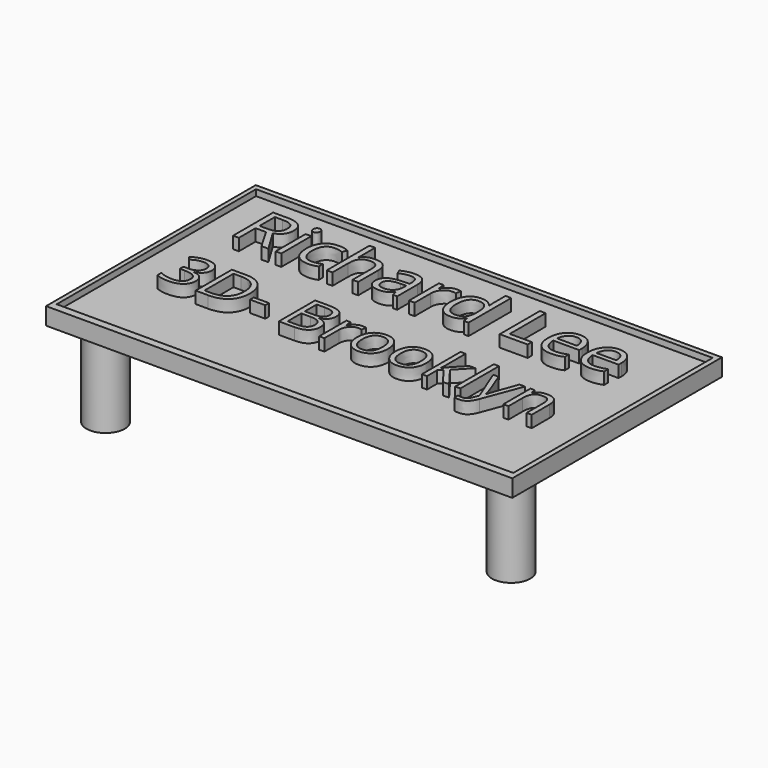
from build123d import *

# Parameters (mm, degrees)
F0_W         = 309.3383610249
F0_H         = 173.9087402821
F1_DEPTH     = 11.43
F2_W         = 303.0182123184
F2_H         = 165.3465926647
F3_DEPTH     = 4.064
F4_TEXT_SIZE = 46.590811384
F7_DEPTH     = 7.874
F5_TEXT_SIZE = 42.1467461758
F8_DEPTH     = 7.874
F10_DEPTH    = 59.436


# Not quite as in the source:
# - Text() gives the source's letters only with a copy of the font that has no kerning and outlines rounded to 1/6400 em; it was checked with that copy


with BuildPart() as f1:
    # F0 (on Top) → F1 (new body)
    with BuildSketch(Plane.XY):
        with Locations((-0.0589936972, 0.3314390779)):
            Rectangle(F0_W, F0_H)
    extrude(amount=F1_DEPTH)

    # F2 (on face) → F3 (cut)
    with BuildSketch(Plane.XY.offset(11.43)):
        with Locations((-0.2423375845, 1.130618155)):
            Rectangle(F2_W, F2_H)
    extrude(amount=-F3_DEPTH, mode=Mode.SUBTRACT)

    # F4 (on face) → F7 (join)
    with BuildSketch(Plane.XY.offset(7.366)):
        with Locations((-128.467800018, 29.9129642029)):
            Text('Richard Lee', F4_TEXT_SIZE, font='Open Sans', text_align=(TextAlign.LEFT, TextAlign.BOTTOM))
    extrude(amount=F7_DEPTH)

    # F5 (on face) → F8 (join)
    with BuildSketch(Plane.XY.offset(7.366)):
        with Locations((-128.7617744142, -30.3456572466)):
            Text('3D- Brooklyn', F5_TEXT_SIZE, font='Open Sans', text_align=(TextAlign.LEFT, TextAlign.BOTTOM))
    extrude(amount=F8_DEPTH)

    # F9 (on face) → F10 (join)
    with BuildSketch(Plane(origin=(0, 0, 0), x_dir=(1, 0, 0), z_dir=(0, 0, -1))):
        with BuildLine():
            Line((134.5220677783, 62.3842328787), (147.2220677783, 62.3842328787))
            ThreePointArc((147.2220677783, 62.3842328787), (134.5220677783, 75.0842328787), (121.8220677783, 62.3842328787))
            Line((121.8220677783, 62.3842328787), (134.5220677783, 62.3842328787))
        make_face()
        with BuildLine():
            ThreePointArc((121.8220677783, 62.3842328787), (134.5220677783, 49.6842328787), (147.2220677783, 62.3842328787))
            Line((147.2220677783, 62.3842328787), (134.5220677783, 62.3842328787))
            Line((134.5220677783, 62.3842328787), (121.8220677783, 62.3842328787))
        make_face()
        with BuildLine():
            ThreePointArc((-147.3367742096, 62.3842328787), (-134.6367742096, 49.6842328787), (-121.9367742096, 62.3842328787))
            Line((-121.9367742096, 62.3842328787), (-134.6367742096, 62.3842328787))
            Line((-134.6367742096, 62.3842328787), (-147.3367742096, 62.3842328787))
        make_face()
        with BuildLine():
            Line((-134.6367742096, 62.3842328787), (-121.9367742096, 62.3842328787))
            ThreePointArc((-121.9367742096, 62.3842328787), (-134.6367742096, 75.0842328787), (-147.3367742096, 62.3842328787))
            Line((-147.3367742096, 62.3842328787), (-134.6367742096, 62.3842328787))
        make_face()
    extrude(amount=F10_DEPTH)


solid = f1.part
